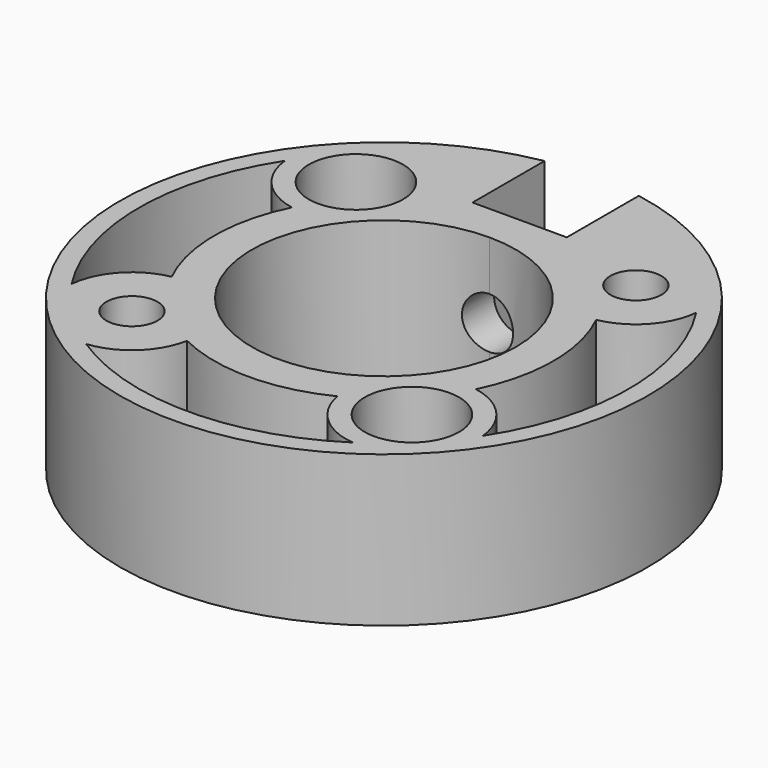
from build123d import *

# Parameters (mm, degrees)
F0_R            = 2.15265
F1_DEPTH        = 12.7
F2_R            = 2.15265
F3_REACH        = 42.6021136501
F6_R            = 3.96875
F7_DEPTH        = 9.525
F9_DEPTH        = 12.7
F9_COPIES_COUNT = 3
F9_COPIES_ANGLE = 180
F10_R           = 3.96875
F11_DEPTH       = 9.525


# Not quite as in the source:
# - a pattern or mirror of a feature is missing from the dataset's text; its kind, count and spacing are read off the source's solid


with BuildPart() as f1:
    # F0 (on Top) → F1 (new body)
    with BuildSketch(Plane.XY):
        with BuildLine():
            Line((3.96875, 14.2875), (0, 14.2875))
            Line((0, 14.2875), (-3.96875, 14.2875))
            Line((-3.96875, 14.2875), (-3.96875, 21.8677764859))
            ThreePointArc((-3.96875, 21.8677764859), (0, -22.225), (3.96875, 21.8677764859))
            Line((3.96875, 21.8677764859), (3.96875, 14.2875))
        make_face()
        with Locations((-11.7865861589, -11.7865861589)):
            Circle(F0_R, mode=Mode.SUBTRACT)
        with Locations((11.7865861589, -11.7865861589)):
            Circle(F0_R, mode=Mode.SUBTRACT)
        with Locations((-11.7865861589, 11.7865861589)):
            Circle(F0_R, mode=Mode.SUBTRACT)
        with BuildLine():
            ThreePointArc((0, 11.1125), (7.8577241059, 7.8577241059), (11.1125, 0))
            ThreePointArc((11.1125, 0), (-7.8577241059, -7.8577241059), (0, 11.1125))
        make_face(mode=Mode.SUBTRACT)
        with Locations((11.7865861589, 11.7865861589)):
            Circle(F0_R, mode=Mode.SUBTRACT)
    extrude(amount=F1_DEPTH)

    f3_end = f1.faces().sort_by_distance((0, -11.1125, 6.35))[0]
    # F2 (on face) → F3 (cut, up to a face of the model that its end follows)
    with BuildSketch(Plane(origin=(0, 14.2875, 0), x_dir=(-1, 0, 0), z_dir=(0, 1, 0))):
        with Locations((0, 6.35)):
            Circle(F2_R)
    f3_long = extrude(amount=-F3_REACH, mode=Mode.PRIVATE)
    add(split(f3_long, bisect_by=f3_end, keep=Keep.ALL, mode=Mode.PRIVATE).solids().sort_by_distance((0, 14.2875, 6.35))[0], mode=Mode.SUBTRACT)

    # F6 (on face) → F7 (cut, through all)
    with BuildSketch(Plane(origin=(0, 0, 0), x_dir=(1, 0, 0), z_dir=(0, 0, -1))):
        with Locations((11.7865861589, -11.7865861589)):
            Circle(F6_R)
        with Locations((-11.7865861589, 11.7865861589)):
            Circle(F6_R)
    extrude(amount=-F7_DEPTH, mode=Mode.SUBTRACT)

    # F8 (on face) → F9 (cut, through all)
    with BuildSketch(Plane(origin=(0, 0, 0), x_dir=(1, 0, 0), z_dir=(0, 0, -1))):
        with BuildLine():
            ThreePointArc((-17.3148424047, -11.229543123), (-15.8788163052, -8.0281867), (-12.8109235396, -6.3255746232))
            ThreePointArc((-12.8109235396, -6.3255746232), (-14.2875, 0), (-12.8109235396, 6.3255746232))
            ThreePointArc((-12.8109235396, 6.3255746232), (-15.8788163052, 8.0281867), (-17.3148424047, 11.229543123))
            ThreePointArc((-17.3148424047, 11.229543123), (-20.6375, 0), (-17.3148424047, -11.229543123))
        make_face()
    f9 = extrude(amount=-F9_DEPTH, mode=Mode.SUBTRACT)

    # F9_copies: F9 ×3 about axis
    f9_copies_axis = Axis((0, 0, 0), (0, 0, 1))
    for i in range(1, F9_COPIES_COUNT):
        add(f9.rotate(f9_copies_axis, i * F9_COPIES_ANGLE / (F9_COPIES_COUNT - 1)), mode=Mode.SUBTRACT)

    # F10 (on face) → F11 (cut, through all)
    with BuildSketch(Plane.XY.offset(12.7)):
        with Locations((11.7865861589, -11.7865861589)):
            Circle(F10_R)
        with Locations((-11.7865861589, 11.7865861589)):
            Circle(F10_R)
    extrude(amount=-F11_DEPTH, mode=Mode.SUBTRACT)


solid = f1.part
